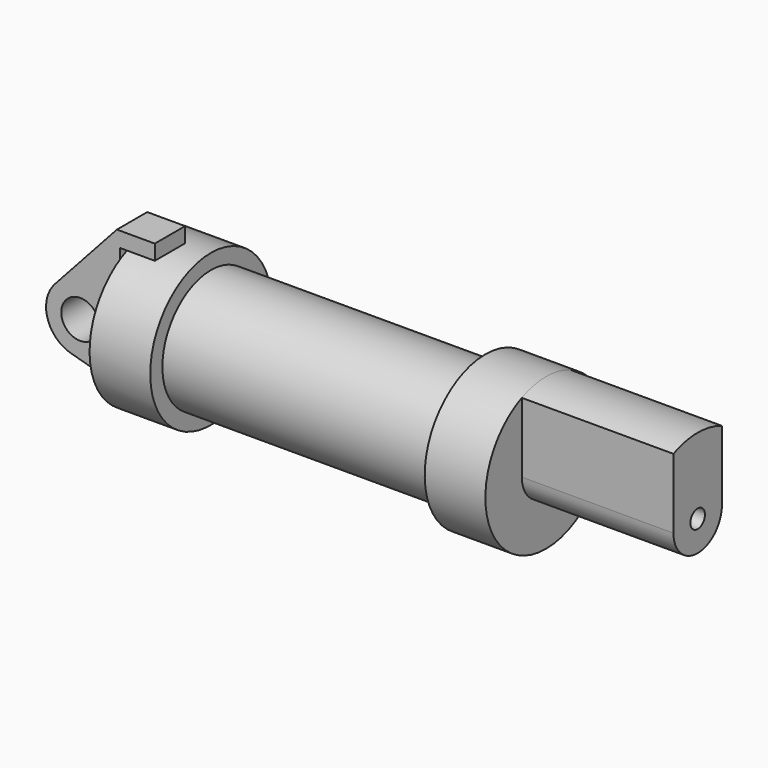
from build123d import *

# Parameters (mm, degrees)
F0_W     = 5.842
F0_H     = 12.7
F0_R     = 3.175
F2_DEPTH = 6.35
F3_R     = 1.524
F4_DEPTH = 25.4


with BuildPart() as f1:
    # F0 (on Front) → F1 (revolve)
    with BuildSketch(Plane.XZ):
        Polygon((5.842, 12.7), (5.842, 0), (66.294, 0), (66.294, 12.7), (56.134, 12.7), (56.134, 10.16), (10.16, 10.16), (10.16, 12.7), align=None)
        with Locations((2.921, 6.35)):
            Rectangle(F0_W, F0_H)
    revolve(axis=Axis((33.147, 0, 0), (-1, 0, 0)))

    # F3 (on face) → F4 (join)
    with BuildSketch(Plane.YZ.offset(66.294)):
        with BuildLine():
            ThreePointArc((-5.079762, -0.049221), (0.024611, -5.07994), (5.08, 0))
            ThreePointArc((5.08, 0), (5.079134, 0.09378), (5.076538, 0.187529))
            Line((5.076538, 0.187529), (5.076538, 11.641253))
            ThreePointArc((5.076538, 11.641253), (-0.001759, 12.7), (-5.079762, 11.639846))
            Line((-5.079762, 11.639846), (-5.079762, -0.049221))
        make_face()
        Circle(F3_R, mode=Mode.SUBTRACT)
    extrude(amount=F4_DEPTH)


with BuildPart() as f2:
    # F0 (on Front) → F2 (new body)
    with BuildSketch(Plane.XZ):
        with BuildLine():
            Line((-0.9398, 0), (0, 0))
            Line((0, 0), (0, 12.7))
            Line((0, 12.7), (5.842, 12.7))
            Line((5.842, 12.7), (5.842, 15.24))
            Line((5.842, 15.24), (-0.508, 15.24))
            Line((-0.508, 15.24), (-10.88063, 3.847543))
            ThreePointArc((-10.88063, 3.847543), (-4.591961, 5.329721), (-0.9398, 0))
        make_face()
        with BuildLine():
            ThreePointArc((-8.182663, -5.506983), (-3.195791, -4.549339), (-0.9398, 0))
            ThreePointArc((-0.9398, 0), (-4.591961, 5.329721), (-10.88063, 3.847543))
            ThreePointArc((-10.88063, 3.847543), (-12.145978, -1.583727), (-8.182663, -5.506983))
        make_face()
        with Locations((-6.6548, 0)):
            Circle(F0_R, mode=Mode.SUBTRACT)
        with BuildLine():
            Line((5.842, 0), (0, 0))
            Line((0, 0), (-0.9398, 0))
            ThreePointArc((-0.9398, 0), (-3.195791, -4.549339), (-8.182663, -5.506983))
            Line((-8.182663, -5.506983), (5.842, -9.398))
            Line((5.842, -9.398), (5.842, 0))
        make_face()
    extrude(amount=F2_DEPTH)


solid = Compound([f1.part, f2.part])
